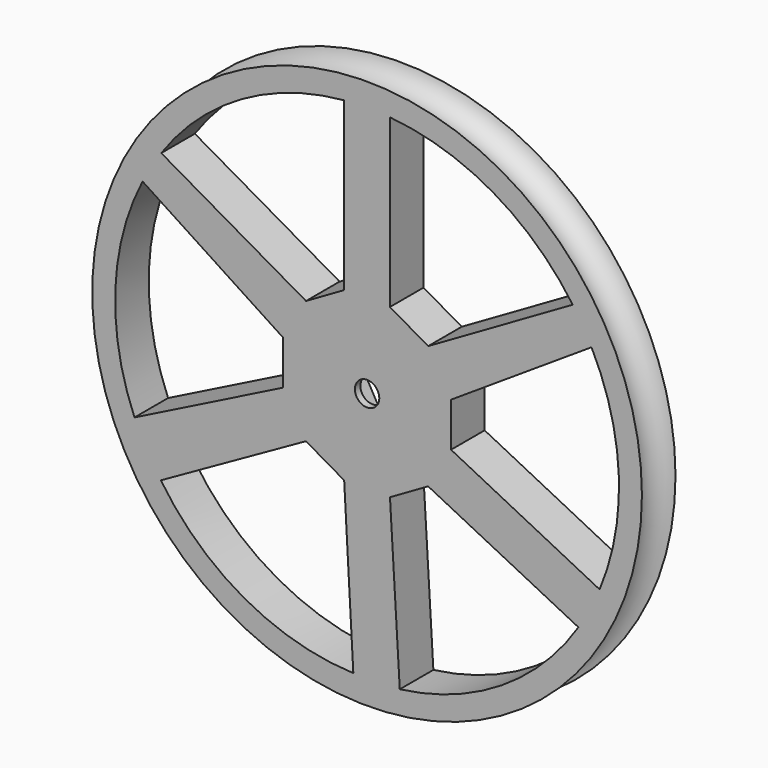
from build123d import *

# Parameters (mm, degrees)
F2_R     = 2.032
F3_DEPTH = 15.875
F4_DEPTH = 10.9982


# Not quite as in the source:
# - a feature names something its author has since deleted; it is built from what else it names


with BuildPart() as f1:
    # F0 (on Top) → F1 (revolve)
    with BuildSketch(Plane.XY):
        with BuildLine():
            Line((0, -5.1666409709), (0, -12.1516409709))
            Line((0, -12.1516409709), (45.72, -12.1516409709))
            ThreePointArc((45.72, -12.1516409709), (42.9147529825, -8.6591409709), (45.72, -5.1666409709))
            Line((45.72, -5.1666409709), (0, -5.1666409709))
        make_face()
    revolve(axis=Axis((0, -8.561744864, 0), (0, 1, 0)))

    # F2 (on Front) → F3 (cut)
    with BuildSketch(Plane.XZ):
        with BuildLine():
            Line((13.97, 3.6661742094), (13.97, -3.6661742094))
            Line((13.97, -3.6661742094), (38.6802071591, -16.0932599922))
            ThreePointArc((38.6802071591, -16.0932599922), (41.8782799617, 1.5705660984), (37.3345500424, 18.9369975174))
            Line((37.3345500424, 18.9369975174), (13.97, 3.6661742094))
        make_face()
        with BuildLine():
            Line((3.81, 41.7094333604), (3.81, 13.9314619955))
            Line((3.81, 13.9314619955), (10.16, 10.2652877862))
            Line((10.16, 10.2652877862), (34.2119266748, 24.1516741264))
            ThreePointArc((34.2119266748, 24.1516741264), (20.9542761873, 36.2954737188), (3.81, 41.7094333604))
        make_face()
        with BuildLine():
            Line((-34.2388233597, 24.0958361272), (-10.16, 10.2652877862))
            Line((-10.16, 10.2652877862), (-3.81, 13.9314619955))
            Line((-3.81, 13.9314619955), (-3.81, 41.7173788368))
            ThreePointArc((-3.81, 41.7173788368), (-20.9781685322, 36.2803485402), (-34.2388233597, 24.0958361272))
        make_face()
        with BuildLine():
            Line((-38.6893950171, -16.0623838358), (-13.97, -3.6661742094))
            Line((-13.97, -3.6661742094), (-13.97, 3.6661742094))
            Line((-13.97, 3.6661742094), (-37.3405062231, 18.9372899969))
            ThreePointArc((-37.3405062231, 18.9372899969), (-41.8787701809, 1.5863648371), (-38.6893950171, -16.0623838358))
        make_face()
        with BuildLine():
            Line((-3.81, -13.9314619955), (-10.16, -10.2652877862))
            Line((-10.16, -10.2652877862), (-34.3038742814, -23.844345572))
            ThreePointArc((-34.3038742814, -23.844345572), (-20.4303998238, -36.5921428083), (-2.2874128339, -41.6726596109))
            Line((-2.2874128339, -41.6726596109), (-3.81, -13.9314619955))
        make_face()
        with BuildLine():
            Line((10.16, -10.2652877862), (3.81, -13.9314619955))
            Line((3.81, -13.9314619955), (5.4400267393, -41.5192010913))
            ThreePointArc((5.4400267393, -41.5192010913), (22.3730839146, -35.4381883413), (35.1536490306, -22.7746857971))
            Line((35.1536490306, -22.7746857971), (10.16, -10.2652877862))
        make_face()
        Circle(F2_R)
    extrude(amount=F3_DEPTH, mode=Mode.SUBTRACT)

    # F2 (on Front) → F4 (cut)
    with BuildSketch(Plane.XZ):
        Polygon((-7.0386894402, 0.071686571), (-3.5814271117, -6.059840579), (3.4572623285, -6.1315271501), (7.0386894402, -0.071686571), (3.5814271117, 6.059840579), (-3.4572623285, 6.1315271501), align=None)
        Circle(F2_R, mode=Mode.SUBTRACT)
    extrude(amount=F4_DEPTH, mode=Mode.SUBTRACT)


solid = f1.part
